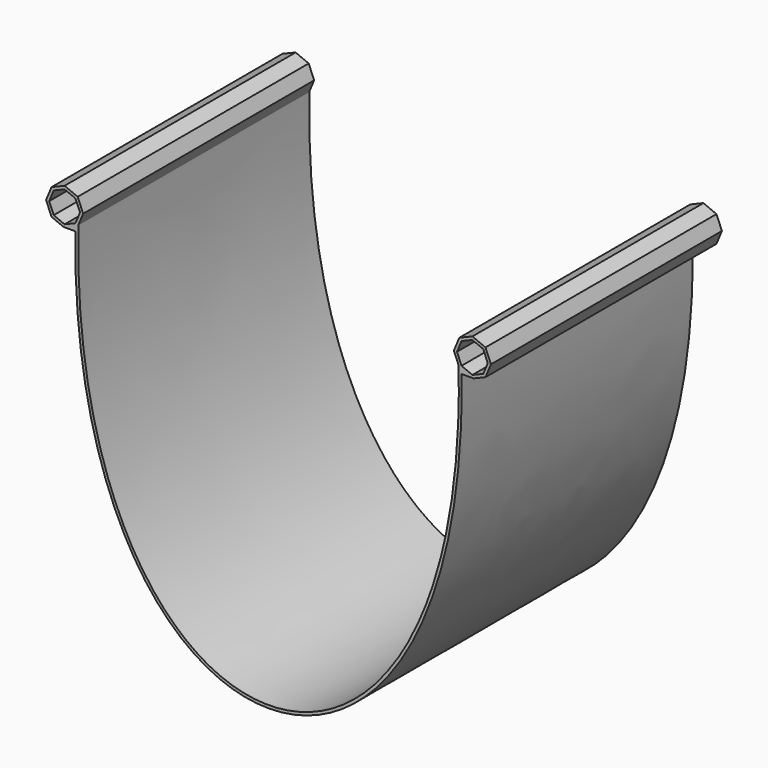
from build123d import *

# Parameters (mm, degrees)
F1_DEPTH = 300
F3_DEPTH = 300


# Not quite as in the source:
# - the dataset's text gives a spline's control points without its knots; the knots are read off the source's solid


with BuildPart() as f1:
    # F0 (on Front) → F1 (new body)
    with BuildSketch(Plane.XZ):
        with BuildLine():
            Line((-424.8167300832, -18.771638081), (-412.4911172581, -18.771638081))
            add(Edge.make_bspline(
                [(-412.4911172581, -18.771638081), (-419.449979951, -513.5140234726), (-4.218700049, -513.5140234726), (-11.1775627419, -18.771638081)],
                knots=[1.9852709954, 1.9852709954, 1.9852709954, 1.9852709954, 399.0559920066, 399.0559920066, 399.0559920066, 399.0559920066], degree=3))
            Line((-11.1775627419, -18.771638081), (1.1480500832, -18.771638081))
            Line((1.1480500832, -18.771638081), (13.6098086653, -13.6098086653))
            Line((13.6098086653, -13.6098086653), (19.2471759958, 0))
            Line((19.2471759958, 0), (13.6098086653, 13.6098086653))
            Line((13.6098086653, 13.6098086653), (-8.39e-08, 19.2471759958))
            Line((-8.39e-08, 19.2471759958), (-13.6098087492, 13.6098086653))
            Line((-13.6098087492, 13.6098086653), (-19.2471760796, 0))
            Line((-19.2471760796, 0), (-14.3005475861, -11.942217597))
            add(Edge.make_bspline(
                [(-409.3681324977, -11.942217597), (-410.7332400225, -74.5841642283), (-402.6757788071, -156.8297634974), (-376.8215805516, -242.8738956774), (-351.1296540078, -295.6294659172), (-320.4812264626, -336.5278862641), (-286.1973466058, -365.615114777), (-249.5756371129, -382.9827448689), (-211.8343400419, -388.7512690899), (-174.093042971, -382.9827448689), (-137.4713334781, -365.615114777), (-103.1874536213, -336.5278862641), (-72.5390260761, -295.6294659172), (-46.8470995323, -242.8738956774), (-20.9929012768, -156.8297634974), (-12.9354400614, -74.5841642283), (-14.3005475861, -11.942217597)],
                knots=[0.000372084, 0.000372084, 0.000372084, 0.000372084, 0.125, 0.1875, 0.25, 0.3125, 0.375, 0.4375, 0.5, 0.5625, 0.625, 0.6875, 0.75, 0.8125, 0.875, 0.999627916, 0.999627916, 0.999627916, 0.999627916], degree=3))
            Line((-409.3681324977, -11.942217597), (-404.4215040042, 0))
            Line((-404.4215040042, 0), (-410.0588713347, 13.6098086653))
            Line((-410.0588713347, 13.6098086653), (-423.66868, 19.2471759958))
            Line((-423.66868, 19.2471759958), (-437.2784886653, 13.6098086653))
            Line((-437.2784886653, 13.6098086653), (-442.9158559958, 0))
            Line((-442.9158559958, 0), (-437.2784886653, -13.6098086653))
            Line((-437.2784886653, -13.6098086653), (-424.8167300832, -18.771638081))
        make_face()
    extrude(amount=F1_DEPTH)

    # F2 (on face) → F3 (cut, symmetric)
    with BuildSketch(Plane.XZ.offset(300)):
        Polygon((-11.313708499, 11.313708499), (-16, 0), (-11.313708499, -11.313708499), (0, -16), (11.313708499, -11.313708499), (16, 0), (11.313708499, 11.313708499), (0, 16), align=None)
        Polygon((-412.354971501, -11.313708499), (-407.66868, 0), (-412.354971501, 11.313708499), (-423.66868, 16), (-434.982388499, 11.313708499), (-439.66868, 0), (-434.982388499, -11.313708499), (-423.66868, -16), align=None)
    extrude(amount=F3_DEPTH, both=True, mode=Mode.SUBTRACT)


solid = f1.part
